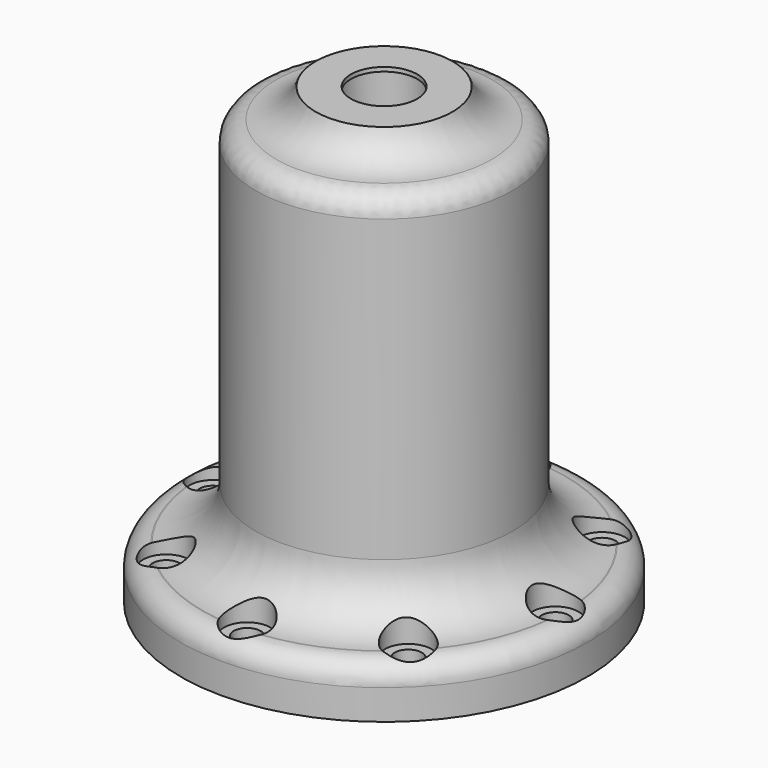
from build123d import *

# Parameters (mm, degrees)
F2_R            = 12.7
F4_R            = 5.08
F3_R            = 3.25
F5_DEPTH        = 25.4
F5_COPIES_COUNT = 8
F7_R            = 5.5626
F8_DEPTH        = 25.4
F8_COPIES_COUNT = 8
F9_R            = 4.7625
F10_DEPTH       = 49.0010001
F11_SIZE2       = 2.6794919243
F11_SIZE        = 10
F13_R           = 5
F14_R           = 2


# Not quite as in the source:
# - a fillet or chamfer that OpenCascade refuses, or shapes differently, is made with other operations: its cross-section is extruded or revolved along the edge and cut away or added
# - a pattern or mirror of a feature is missing from the dataset's text; its kind, count and spacing are read off the source's solid


with BuildPart() as f1:
    # F0 (on Right) → F1 (revolve)
    with BuildSketch(Plane.YZ):
        Polygon((-29, 0), (-25, 0), (-25, 88), (-12.5, 88), (-12.5, 95), (-8, 95), (-8, 96), (-9, 96), (-9, 104), (-8, 104), (-8, 105), (-16.5, 105), (-16.5, 98), (-31, 98), (-31, 8), (-49, 8), (-49, -4.35), (-37, -4.35), (-37, 2), (-29, 2), align=None)
    revolve(axis=Axis((0, 0, 24.2049096316), (0, 0, 1)))

    # F2
    f2_edges = [f1.edges().sort_by_distance(p)[0] for p in [
        (0, 31, 8),
    ]]
    fillet(f2_edges, radius=F2_R)

    # F4
    f4_edges = [f1.edges().sort_by_distance(p)[0] for p in [
        (0, 49, 8),
    ]]
    fillet(f4_edges, radius=F4_R)

    # F3 (on face) → F5 (cut)
    with BuildSketch(Plane(origin=(0, 0, -4.35), x_dir=(1, 0, 0), z_dir=(0, 0, -1))):
        with Locations((41.275, 0)):
            Circle(F3_R)
    f5 = extrude(amount=-F5_DEPTH, mode=Mode.SUBTRACT)

    # F5_copies: F5 ×8 about axis
    f5_copies_axis = Axis((0, 0, 0), (0, 0, 1))
    for i in range(1, F5_COPIES_COUNT):
        add(f5.rotate(f5_copies_axis, i * 360 / F5_COPIES_COUNT), mode=Mode.SUBTRACT)

    # F7 (on offset) → F8 (cut)
    with BuildSketch(Plane(origin=(0, 0, 5.175), x_dir=(1, 0, 0), z_dir=(0, 0, -1))):
        with Locations((41.275, 0)):
            Circle(F7_R)
    f8 = extrude(amount=-F8_DEPTH, mode=Mode.SUBTRACT)

    # F8_copies: F8 ×8 about axis
    f8_copies_axis = Axis((0, 0, 0), (0, 0, 1))
    for i in range(1, F8_COPIES_COUNT):
        add(f8.rotate(f8_copies_axis, i * 360 / F8_COPIES_COUNT), mode=Mode.SUBTRACT)

    # F9 (on Front) → F10 (cut, through all)
    with BuildSketch(Plane.XZ):
        with Locations((0, 62.611)):
            Circle(F9_R)
    extrude(amount=-F10_DEPTH, mode=Mode.SUBTRACT)

    # F11
    f11_edges = [f1.edges().sort_by_distance(p)[0] for p in [
        (0, 25, 0),
    ]]
    chamfer(f11_edges, length=F11_SIZE, length2=F11_SIZE2)

    # F12: fillet of radius 10 on 1 edges, made by hand

    # F12_s1 → F12_t2 (revolve)
    with BuildSketch(Plane.YZ):
        with BuildLine():
            ThreePointArc((-26.0393920142, 98), (-20.1233122311, 99.9377422517), (-16.5, 105))
            Line((-16.5, 105), (-16.5, 98))
            Line((-16.5, 98), (-26.0393920142, 98))
        make_face()
    revolve(axis=Axis((0, 0, 98), (0, 0, 1)))

    # F13
    f13_edges = [f1.edges().sort_by_distance(p)[0] for p in [
        (0, 31, 98),
    ]]
    fillet(f13_edges, radius=F13_R)

    # F14
    f14_edges = [f1.edges().sort_by_distance(p)[0] for p in [
        (0, 25, 88),
    ]]
    fillet(f14_edges, radius=F14_R)


solid = f1.part
